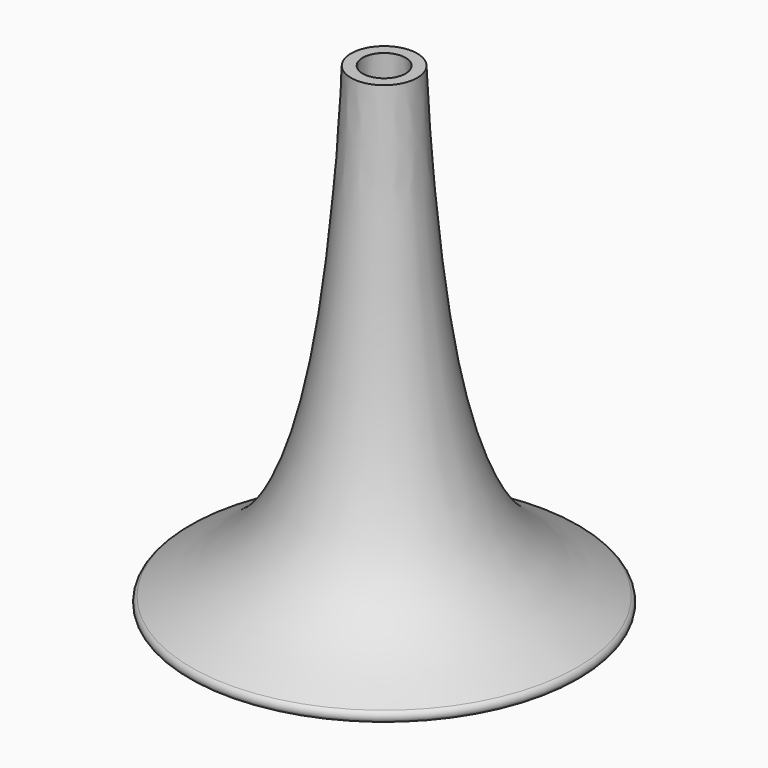
from build123d import *


# Not quite as in the source:
# - the dataset's text gives a spline's control points without its knots; the knots are read off the source's solid


with BuildPart() as f1:
    # F0 (on Front) → F1 (revolve)
    with BuildSketch(Plane.XZ):
        with BuildLine():
            add(Edge.make_bspline(
                [(40.8965982497, 0), (33.1633556054, 4.1185675105), (14.8508325851, 13.8714442552), (6.5557692481, 66.5664577266), (5.2787821832, 92.0605652909), (4.682819359, 103.9585247636)],
                knots=[0, 0, 0, 0, 0.2804904807, 0.6642088734, 1, 1, 1, 1], degree=3))
            ThreePointArc((40.8965982497, 0), (42.6145261991, 0.5239496211), (42.090576578, 2.2418775706))
            add(Edge.make_bspline(
                [(42.090576578, 2.2418775706), (40.3674248186, 3.159593098), (36.9642017907, 4.9728446594), (32.1338664363, 7.9144799924), (28.44067819, 10.7774176375), (25.7291958678, 13.4575786399), (24.1428280505, 15.3284506058), (22.9429657646, 16.9649101865), (22.0801981067, 18.266143088), (21.2513895254, 19.6541794499), (20.187878668, 21.6209207611), (18.9395888059, 24.2810392017), (17.1145626752, 28.9128131349), (15.1499951443, 35.2997042967), (13.2529808532, 43.5845770609), (12.0034160078, 50.7336217676), (11.1678084816, 56.4401514937), (10.6140321501, 60.6738663199), (10.1241221968, 64.8238089953), (9.6884800665, 68.8449688441), (9.3019131289, 72.7326282006), (8.8454305294, 77.7617318227), (8.3729320865, 83.789471924), (7.9234747699, 90.7172131214), (7.5522000665, 97.4463631801), (7.3305639626, 101.8710540131), (7.2196388262, 104.0855927787)],
                knots=[0, 0, 0, 0, 0.0625, 0.125, 0.1875, 0.21875, 0.25, 0.265625, 0.28125, 0.296875, 0.3125, 0.34375, 0.375, 0.4375, 0.5, 0.5625, 0.59375, 0.625, 0.65625, 0.6875, 0.71875, 0.75, 0.8125, 0.875, 0.9375, 1, 1, 1, 1], degree=3))
            Line((7.2196388262, 104.0855927787), (4.682819359, 104.0855927787))
            Line((4.682819359, 104.0855927787), (4.682819359, 103.9585247636))
        make_face()
    revolve(axis=Axis((0, 0, 52.7466833591), (0, 0, 1)))


solid = f1.part
